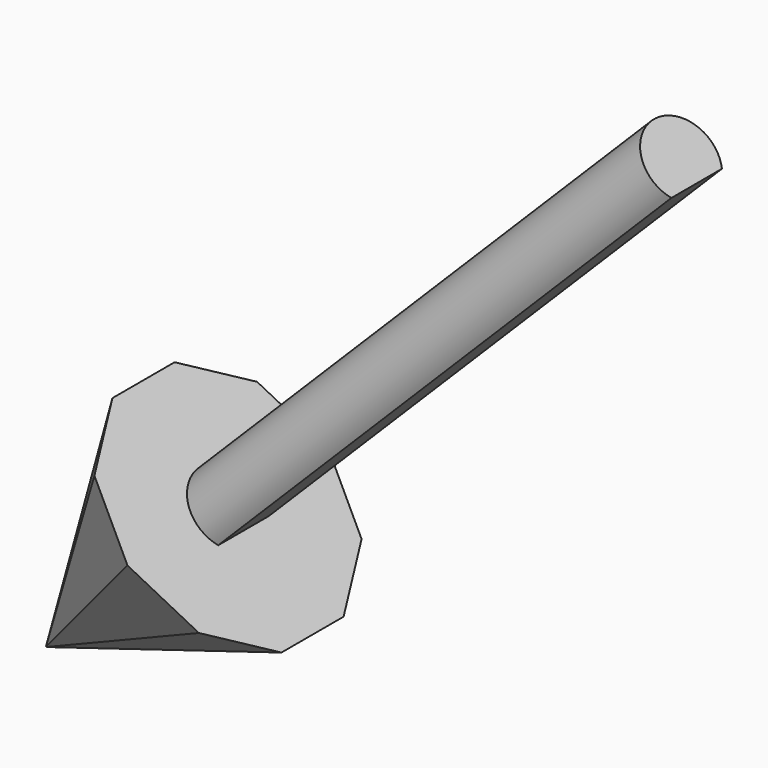
from build123d import *

# Parameters (mm, degrees)
F7_DEPTH = 50
F8_W     = 5
F8_H     = 5
F9_DEPTH = 12.5


with BuildPart() as f5:
    # F2 (on face) → F5 section 0
    with BuildSketch(Plane(origin=(14.1421356237, 0, 14.1421356237), x_dir=(0.7071067812, 0, -0.7071067812), z_dir=(-0.7071067812, 0, -0.7071067812))):
        Polygon((-9.3261531631, 3.0302508528), (-9.3261531631, -3.0302508528), (-5.7638796391, -7.933299727), (0, -9.8060977485), (5.7638796391, -7.933299727), (9.3261531631, -3.0302508528), (9.3261531631, 3.0302508528), (5.7638796391, 7.933299727), (0, 9.8060977485), (-5.7638796391, 7.933299727), align=None)
    # F4 (on face) → F5 section 1
    with BuildSketch(Plane(origin=(0, 0, 0), x_dir=(0.7071067812, 0, -0.7071067812), z_dir=(-0.7071067812, 0, -0.7071067812))):
        Polygon((-0.0475528258, 0.0154508497), (-0.0475528258, -0.0154508497), (-0.0293892626, -0.0404508497), (0, -0.05), (0.0293892626, -0.0404508497), (0.0475528258, -0.0154508497), (0.0475528258, 0.0154508497), (0.0293892626, 0.0404508497), (0, 0.05), (-0.0293892626, 0.0404508497), align=None)
    loft()

    # F6 (on face) → F7 (join)
    with BuildSketch(Plane(origin=(14.1421356237, 0, 14.1421356237), x_dir=(0.7071067812, 0, -0.7071067812), z_dir=(0.7071067812, 0, 0.7071067812))):
        with BuildLine():
            Line((1.7084597584, -2.4660018763), (1.7084597584, 2.4660018763))
            ThreePointArc((1.7084597584, 2.4660018763), (-3, 0), (1.7084597584, -2.4660018763))
        make_face()
    extrude(amount=F7_DEPTH)

    # F8 (on Front) → F9 (cut, symmetric)
    with BuildSketch(Plane.XZ):
        with Locations((11.3405170292, 22.6421356237)):
            Rectangle(F8_W, F8_H)
    extrude(amount=F9_DEPTH, both=True, mode=Mode.SUBTRACT)


solid = f5.part
